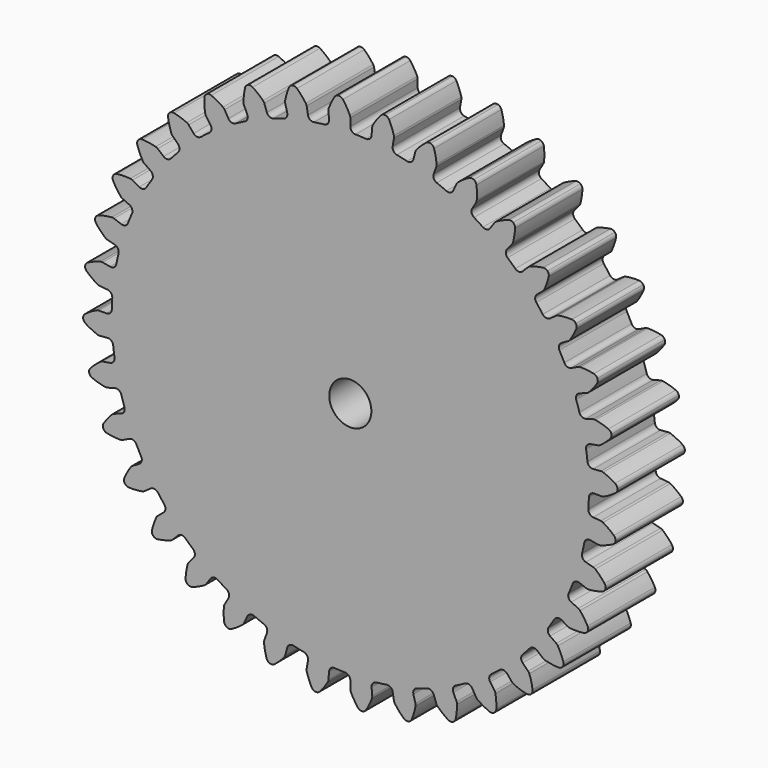
from build123d import *

# Parameters (mm, degrees)
F0_R     = 3.175
F1_DEPTH = 12.7


# Not quite as in the source:
# - ends of sketch curves that miss each other by under 0.0002 mm in the source are joined


with BuildPart() as f1:
    # F0 (on Front) → F1 (new body)
    with BuildSketch(Plane.XZ):
        with BuildLine():
            ThreePointArc((-3.2042183364, 36.6243831745), (-3.3814286726, 36.051583162), (-3.9087160554, 35.7661512552))
            ThreePointArc((-3.9087160554, 35.7661512552), (-4.6962149225, 35.6712938119), (-5.4814313293, 35.5590993614))
            ThreePointArc((-5.4814313293, 35.5590993614), (-6.0646270438, 35.6983333949), (-6.3840506365, 36.2057503103))
            Line((-6.3840506365, 36.2057503103), (-6.5860311993, 37.3512390039))
            ThreePointArc((-6.5860311993, 37.3512390039), (-6.634615599, 37.5176976448), (-6.7181878779, 37.6696338066))
            ThreePointArc((-6.7181878779, 37.6696338066), (-7.3438117619, 38.466585852), (-8.0505487137, 39.1925753064))
            ThreePointArc((-8.0505487137, 39.1925753064), (-8.3662011151, 39.3676879642), (-8.7270294051, 39.3778774973))
            ThreePointArc((-8.7270294051, 39.3778774973), (-8.7297356308, 39.3772929981), (-8.7324354314, 39.3766790101))
            ThreePointArc((-8.7324354314, 39.3766790101), (-9.0551506376, 39.2149515322), (-9.26722306, 38.9228450977))
            ThreePointArc((-9.26722306, 38.9228450977), (-9.6009278616, 37.9661952598), (-9.8311291712, 36.9795113367))
            ThreePointArc((-9.8311291712, 36.9795113367), (-9.8426603818, 36.806491239), (-9.8163443401, 36.6350958219))
            Line((-9.8163443401, 36.6350958219), (-9.5152964565, 35.5115698246))
            ThreePointArc((-9.5152964565, 35.5115698246), (-9.5903488911, 34.9166996794), (-10.0600608633, 34.5440416315))
            ThreePointArc((-10.0600608633, 34.5440416315), (-10.8191240309, 34.3138775427), (-11.5729288743, 34.0670361799))
            ThreePointArc((-11.5729288743, 34.0670361799), (-12.1714422717, 34.1028840626), (-12.5741251249, 34.54712485))
            Line((-12.5741251249, 34.54712485), (-12.9719491733, 35.6401374398))
            ThreePointArc((-12.9719491733, 35.6401374398), (-13.0487007064, 35.7956306075), (-13.1573867722, 35.9307463436))
            ThreePointArc((-13.1573867722, 35.9307463436), (-13.911895294, 36.6069524494), (-14.7339620693, 37.1991889089))
            ThreePointArc((-14.7339620693, 37.1991889089), (-15.0752269954, 37.3168287477), (-15.4323428867, 37.2642063038))
            ThreePointArc((-15.4323428867, 37.2642063038), (-15.4349065016, 37.2631607534), (-15.4374586682, 37.2620872777))
            ThreePointArc((-15.4374586682, 37.2620872777), (-15.7271874235, 37.0467778962), (-15.8853142392, 36.7222832251))
            ThreePointArc((-15.8853142392, 36.7222832251), (-16.047828814, 35.7222198171), (-16.1031969833, 34.710551802))
            ThreePointArc((-16.1031969833, 34.710551802), (-16.0845083842, 34.5381578946), (-16.0288296405, 34.3739360918))
            Line((-16.0288296405, 34.3739360918), (-15.5372571087, 33.3197553953))
            ThreePointArc((-15.5372571087, 33.3197553953), (-15.5078712115, 32.7208899458), (-15.9057358125, 32.2723287829))
            ThreePointArc((-15.9057358125, 32.2723287829), (-16.6132995304, 31.913851468), (-17.3127888316, 31.5398633428))
            ThreePointArc((-17.3127888316, 31.5398633428), (-17.9084343851, 31.4712358548), (-18.3821411842, 31.8388024829))
            Line((-18.3821411842, 31.8388024829), (-18.9637210357, 32.8461283345))
            ThreePointArc((-18.9637210357, 32.8461283345), (-19.0663076459, 32.9859314476), (-19.1968051274, 33.1001213348))
            ThreePointArc((-19.1968051274, 33.1001213348), (-20.0572729274, 33.6350353206), (-20.9696914432, 34.0755239801))
            ThreePointArc((-20.9696914432, 34.0755239801), (-21.3261997318, 34.1321165729), (-21.6687524388, 34.0182810585))
            ThreePointArc((-21.6687524388, 34.0182810585), (-21.6710955487, 34.0168062252), (-21.6734225351, 34.015305879))
            ThreePointArc((-21.6734225351, 34.015305879), (-21.9213615778, 33.7529566604), (-22.0207381836, 33.4059333591))
            ThreePointArc((-22.0207381836, 33.4059333591), (-22.0071246085, 32.3928428016), (-21.8859773037, 31.3869297152))
            ThreePointArc((-21.8859773037, 31.3869297152), (-21.8376367385, 31.2204000998), (-21.7542870633, 31.0683417075))
            Line((-21.7542870633, 31.0683417075), (-21.0871260658, 30.1155370589))
            ThreePointArc((-21.0871260658, 30.1155370589), (-20.9541947126, 29.5308725287), (-21.2681230277, 29.0200375549))
            ThreePointArc((-21.2681230277, 29.0200375549), (-21.9026883304, 28.5441391657), (-22.526608461, 28.054367718))
            ThreePointArc((-22.526608461, 28.054367718), (-23.1012877819, 27.8833500709), (-23.6316251854, 28.1630742135))
            Line((-23.6316251854, 28.1630742135), (-24.3792898306, 29.0541062406))
            ThreePointArc((-24.3792898306, 29.0541062406), (-24.5045944755, 29.1739714524), (-24.6529382729, 29.2637658888))
            ThreePointArc((-24.6529382729, 29.2637658888), (-25.5932204724, 29.6411346638), (-26.5682673537, 29.9164914982))
            ThreePointArc((-26.5682673537, 29.9164914982), (-26.929186681, 29.9103173077), (-27.246767913, 29.7387275572))
            ThreePointArc((-27.246767913, 29.7387275572), (-27.2488193237, 29.7368682532), (-27.2508504255, 29.7349866237))
            ThreePointArc((-27.2508504255, 29.7349866237), (-27.4494662534, 29.4335689163), (-27.4870731413, 29.0745611122))
            ThreePointArc((-27.4870731413, 29.0745611122), (-27.2977450579, 28.0792256492), (-27.0037632785, 27.1096316515))
            ThreePointArc((-27.0037632785, 27.1096316515), (-26.9272395509, 26.9540262462), (-26.8187514818, 26.8187514818))
            Line((-26.8187514818, 26.8187514818), (-25.9962733681, 25.9962733681))
            ThreePointArc((-25.9962733681, 25.9962733681), (-25.7638356106, 25.4435744931), (-25.984289087, 24.8859871706))
            ThreePointArc((-25.984289087, 24.8859871706), (-26.5265750288, 24.3071276388), (-27.0559684913, 23.7164543263))
            ThreePointArc((-27.0559684913, 23.7164543263), (-27.5922202392, 23.4482428047), (-28.1630742135, 23.6316251854))
            Line((-28.1630742135, 23.6316251854), (-29.0541062406, 24.3792898306))
            ThreePointArc((-29.0541062406, 24.3792898306), (-29.1983216019, 24.4755750974), (-29.360004364, 24.5382457244))
            ThreePointArc((-29.360004364, 24.5382457244), (-30.3515309641, 24.7466031293), (-31.3595799049, 24.8484615606))
            ThreePointArc((-31.3595799049, 24.8484615606), (-31.7139439196, 24.7797081865), (-31.9969041317, 24.5555778676))
            ThreePointArc((-31.9969041317, 24.5555778676), (-31.9986015121, 24.5533905869), (-32.0002750154, 24.5511848465))
            ThreePointArc((-32.0002750154, 24.5511848465), (-32.1435327869, 24.2198570747), (-32.1182272908, 23.8597730383))
            ThreePointArc((-32.1182272908, 23.8597730383), (-31.7589373371, 22.9124354342), (-31.3010535707, 22.0086211482))
            ThreePointArc((-31.3010535707, 22.0086211482), (-31.1986718154, 21.8686679446), (-31.0683417075, 21.7542870633))
            Line((-31.0683417075, 21.7542870633), (-30.1155370589, 21.0871260658))
            ThreePointArc((-30.1155370589, 21.0871260658), (-29.7906554007, 20.5831863217), (-29.910935671, 19.995788659))
            ThreePointArc((-29.910935671, 19.995788659), (-30.344465168, 19.3315563387), (-30.7632466099, 18.6579284709))
            ThreePointArc((-30.7632466099, 18.6579284709), (-31.2447770469, 18.3006725462), (-31.8388024829, 18.3821411842))
            Line((-31.8388024829, 18.3821411842), (-32.8461283345, 18.9637210357))
            ThreePointArc((-32.8461283345, 18.9637210357), (-33.0048725015, 19.0335007782), (-33.1749815793, 19.0671433806))
            ThreePointArc((-33.1749815793, 19.0671433806), (-34.1876255461, 19.1001585812), (-35.1980474894, 19.0254236925))
            ThreePointArc((-35.1980474894, 19.0254236925), (-35.5350890203, 18.8961801711), (-35.7748306096, 18.6263193703))
            ThreePointArc((-35.7748306096, 18.6263193703), (-35.7761223856, 18.6238705723), (-35.7773874418, 18.6214077412))
            ThreePointArc((-35.7773874418, 18.6214077412), (-35.8609343421, 18.2702371318), (-35.7734853566, 17.9200178343))
            ThreePointArc((-35.7734853566, 17.9200178343), (-35.255150376, 17.0494624628), (-34.6472771892, 16.2388898283))
            ThreePointArc((-34.6472771892, 16.2388898283), (-34.5221482241, 16.1188412335), (-34.3739360918, 16.0288296405))
            Line((-34.3739360918, 16.0288296405), (-33.3197553953, 15.5372571087))
            ThreePointArc((-33.3197553953, 15.5372571087), (-32.9123012013, 15.0973884495), (-32.9287536103, 14.4980282274))
            ThreePointArc((-32.9287536103, 14.4980282274), (-33.2403540882, 13.7686054814), (-33.5357990473, 13.0324909004))
            ThreePointArc((-33.5357990473, 13.0324909004), (-33.9479771147, 12.597045613), (-34.54712485, 12.5741251249))
            Line((-34.54712485, 12.5741251249), (-35.6401374398, 12.9719491733))
            ThreePointArc((-35.6401374398, 12.9719491733), (-35.8085870514, 13.0131031693), (-35.9819537667, 13.0166955336))
            ThreePointArc((-35.9819537667, 13.0166955336), (-36.9849464257, 12.8733653796), (-37.967040212, 12.6243079527))
            ThreePointArc((-37.967040212, 12.6243079527), (-38.2765184228, 12.4385012832), (-38.4657569623, 12.1311095843))
            ThreePointArc((-38.4657569623, 12.1311095843), (-38.4666038841, 12.1284736744), (-38.4674220551, 12.1258285845))
            ThreePointArc((-38.4674220551, 12.1258285845), (-38.4887195539, 11.7654852788), (-38.3417841721, 11.4357719564))
            ThreePointArc((-38.3417841721, 11.4357719564), (-37.6801535108, 10.6684502019), (-36.9407608227, 9.9757480582))
            ThreePointArc((-36.9407608227, 9.9757480582), (-36.796686628, 9.879251688), (-36.6350958219, 9.8163443401))
            Line((-36.6350958219, 9.8163443401), (-35.5115698246, 9.5152964565))
            ThreePointArc((-35.5115698246, 9.5152964565), (-35.0339233843, 9.1528640689), (-34.9460480339, 8.5597525445))
            ThreePointArc((-34.9460480339, 8.5597525445), (-35.1262516698, 7.7873025138), (-35.2893832006, 7.0110676886))
            ThreePointArc((-35.2893832006, 7.0110676886), (-35.6196850763, 6.5106638233), (-36.2057503103, 6.3840506365))
            Line((-36.2057503103, 6.3840506365), (-37.3512390039, 6.5860311993))
            ThreePointArc((-37.3512390039, 6.5860311993), (-37.5242758038, 6.5973090056), (-37.6956324966, 6.5707419796))
            ThreePointArc((-37.6956324966, 6.5707419796), (-38.6584984233, 6.2554214853), (-39.58242363, 5.839609004))
            ThreePointArc((-39.58242363, 5.839609004), (-39.8549351818, 5.602884828), (-39.9879207543, 5.2673021721))
            ThreePointArc((-39.9879207543, 5.2673021721), (-39.9882970885, 5.2645592413), (-39.9886435147, 5.2618122623))
            ThreePointArc((-39.9886435147, 5.2618122623), (-39.9470444982, 4.9032451093), (-39.7450872775, 4.6040559343))
            ThreePointArc((-39.7450872775, 4.6040559343), (-38.9602642482, 3.9632824801), (-38.1118181316, 3.4094982313))
            ThreePointArc((-38.1118181316, 3.4094982313), (-37.9531763288, 3.3394860792), (-37.7831167038, 3.3055943843))
            Line((-37.7831167038, 3.3055943843), (-36.6243831745, 3.2042183364))
            ThreePointArc((-36.6243831745, 3.2042183364), (-36.0910575332, 2.9302345451), (-35.9015244715, 2.3613931119))
            ThreePointArc((-35.9015244715, 2.3613931119), (-35.9448558691, 1.5693863), (-35.9707173026, 0.7766167329))
            ThreePointArc((-35.9707173026, 0.7766167329), (-36.2091069313, 0.2264588079), (-36.7642823684, 0))
            Line((-36.7642823684, 0), (-37.9274420715, 0))
            ThreePointArc((-37.9274420715, 0), (-38.0998084241, -0.0189410539), (-38.263948508, -0.0748602444))
            ThreePointArc((-38.263948508, -0.0748602444), (-39.1574315086, -0.5525902255), (-39.9951151356, -1.1225235092))
            ThreePointArc((-39.9951151356, -1.1225235092), (-40.2223799029, -1.4029724475), (-40.2950718091, -1.7565495511))
            ThreePointArc((-40.2950718091, -1.7565495511), (-40.294966121, -1.7593161604), (-40.2948302763, -1.7620815628))
            ThreePointArc((-40.2948302763, -1.7620815628), (-40.1915987096, -2.1079776817), (-39.9407560179, -2.3675519975))
            ThreePointArc((-39.9407560179, -2.3675519975), (-39.0565870713, -2.8623075744), (-38.124867132, -3.2603474741))
            ThreePointArc((-38.124867132, -3.2603474741), (-37.956477972, -3.3017481243), (-37.7831167038, -3.3055943843))
            Line((-37.7831167038, -3.3055943843), (-36.6243831745, -3.2042183364))
            ThreePointArc((-36.6243831745, -3.2042183364), (-36.051583162, -3.3814286726), (-35.7661512552, -3.9087160554))
            ThreePointArc((-35.7661512552, -3.9087160554), (-35.6712938119, -4.6962149225), (-35.5590993614, -5.4814313293))
            ThreePointArc((-35.5590993614, -5.4814313293), (-35.6983333949, -6.0646270438), (-36.2057503103, -6.3840506365))
            Line((-36.2057503103, -6.3840506365), (-37.3512390039, -6.5860311993))
            ThreePointArc((-37.3512390039, -6.5860311993), (-37.5176976448, -6.634615599), (-37.6696338066, -6.7181878779))
            ThreePointArc((-37.6696338066, -6.7181878779), (-38.466585852, -7.3438117619), (-39.1925753064, -8.0505487137))
            ThreePointArc((-39.1925753064, -8.0505487137), (-39.3676879642, -8.3662011151), (-39.3778774973, -8.7270294051))
            ThreePointArc((-39.3778774973, -8.7270294051), (-39.3772929981, -8.7297356308), (-39.3766790101, -8.7324354314))
            ThreePointArc((-39.3766790101, -8.7324354314), (-39.2149515322, -9.0551506376), (-38.9228450977, -9.26722306))
            ThreePointArc((-38.9228450977, -9.26722306), (-37.9661952598, -9.6009278616), (-36.9795113367, -9.8311291712))
            ThreePointArc((-36.9795113367, -9.8311291712), (-36.806491239, -9.8426603818), (-36.6350958219, -9.8163443401))
            Line((-36.6350958219, -9.8163443401), (-35.5115698246, -9.5152964565))
            ThreePointArc((-35.5115698246, -9.5152964565), (-34.9166996794, -9.5903488911), (-34.5440416315, -10.0600608633))
            ThreePointArc((-34.5440416315, -10.0600608633), (-34.3138775427, -10.8191240309), (-34.0670361799, -11.5729288743))
            ThreePointArc((-34.0670361799, -11.5729288743), (-34.1028840626, -12.1714422717), (-34.54712485, -12.5741251249))
            Line((-34.54712485, -12.5741251249), (-35.6401374398, -12.9719491733))
            ThreePointArc((-35.6401374398, -12.9719491733), (-35.7956306075, -13.0487007064), (-35.9307463436, -13.1573867722))
            ThreePointArc((-35.9307463436, -13.1573867722), (-36.6069524494, -13.911895294), (-37.1991889089, -14.7339620693))
            ThreePointArc((-37.1991889089, -14.7339620693), (-37.3168287477, -15.0752269954), (-37.2642063038, -15.4323428867))
            ThreePointArc((-37.2642063038, -15.4323428867), (-37.2631607534, -15.4349065016), (-37.2620872777, -15.4374586682))
            ThreePointArc((-37.2620872777, -15.4374586682), (-37.0467778962, -15.7271874235), (-36.7222832251, -15.8853142392))
            ThreePointArc((-36.7222832251, -15.8853142392), (-35.7222198171, -16.047828814), (-34.710551802, -16.1031969833))
            ThreePointArc((-34.710551802, -16.1031969833), (-34.5381578946, -16.0845083842), (-34.3739360918, -16.0288296405))
            Line((-34.3739360918, -16.0288296405), (-33.3197553953, -15.5372571087))
            ThreePointArc((-33.3197553953, -15.5372571087), (-32.7208899458, -15.5078712115), (-32.2723287829, -15.9057358125))
            ThreePointArc((-32.2723287829, -15.9057358125), (-31.913851468, -16.6132995304), (-31.5398633428, -17.3127888316))
            ThreePointArc((-31.5398633428, -17.3127888316), (-31.4712358548, -17.9084343851), (-31.8388024829, -18.3821411842))
            Line((-31.8388024829, -18.3821411842), (-32.8461283345, -18.9637210357))
            ThreePointArc((-32.8461283345, -18.9637210357), (-32.9859314476, -19.0663076459), (-33.1001213348, -19.1968051274))
            ThreePointArc((-33.1001213348, -19.1968051274), (-33.6350353206, -20.0572729274), (-34.0755239801, -20.9696914432))
            ThreePointArc((-34.0755239801, -20.9696914432), (-34.1321165729, -21.3261997318), (-34.0182810585, -21.6687524388))
            ThreePointArc((-34.0182810585, -21.6687524388), (-34.0168062252, -21.6710955487), (-34.015305879, -21.6734225351))
            ThreePointArc((-34.015305879, -21.6734225351), (-33.7529566604, -21.9213615778), (-33.4059333591, -22.0207381836))
            ThreePointArc((-33.4059333591, -22.0207381836), (-32.3928428016, -22.0071246085), (-31.3869297152, -21.8859773037))
            ThreePointArc((-31.3869297152, -21.8859773037), (-31.2204000998, -21.8376367385), (-31.0683417075, -21.7542870633))
            Line((-31.0683417075, -21.7542870633), (-30.1155370589, -21.0871260658))
            ThreePointArc((-30.1155370589, -21.0871260658), (-29.5308725287, -20.9541947126), (-29.0200375549, -21.2681230277))
            ThreePointArc((-29.0200375549, -21.2681230277), (-28.5441391657, -21.9026883304), (-28.054367718, -22.526608461))
            ThreePointArc((-28.054367718, -22.526608461), (-27.8833500709, -23.1012877819), (-28.1630742135, -23.6316251854))
            Line((-28.1630742135, -23.6316251854), (-29.0541062406, -24.3792898306))
            ThreePointArc((-29.0541062406, -24.3792898306), (-29.1739714524, -24.5045944755), (-29.2637658888, -24.6529382729))
            ThreePointArc((-29.2637658888, -24.6529382729), (-29.6411346638, -25.5932204724), (-29.9164914982, -26.5682673537))
            ThreePointArc((-29.9164914982, -26.5682673537), (-29.9103173077, -26.929186681), (-29.7387275572, -27.246767913))
            ThreePointArc((-29.7387275572, -27.246767913), (-29.7368682532, -27.2488193237), (-29.7349866237, -27.2508504255))
            ThreePointArc((-29.7349866237, -27.2508504255), (-29.4335689163, -27.4494662534), (-29.0745611122, -27.4870731413))
            ThreePointArc((-29.0745611122, -27.4870731413), (-28.0792256492, -27.2977450579), (-27.1096316515, -27.0037632785))
            ThreePointArc((-27.1096316515, -27.0037632785), (-26.9540262462, -26.9272395509), (-26.8187514818, -26.8187514818))
            Line((-26.8187514818, -26.8187514818), (-25.9962733681, -25.9962733681))
            ThreePointArc((-25.9962733681, -25.9962733681), (-25.4435744931, -25.7638356106), (-24.8859871706, -25.984289087))
            ThreePointArc((-24.8859871706, -25.984289087), (-24.3071276388, -26.5265750288), (-23.7164543263, -27.0559684913))
            ThreePointArc((-23.7164543263, -27.0559684913), (-23.4482428047, -27.5922202392), (-23.6316251854, -28.1630742135))
            Line((-23.6316251854, -28.1630742135), (-24.3792898306, -29.0541062406))
            ThreePointArc((-24.3792898306, -29.0541062406), (-24.4755750974, -29.1983216019), (-24.5382457244, -29.360004364))
            ThreePointArc((-24.5382457244, -29.360004364), (-24.7466031293, -30.3515309641), (-24.8484615606, -31.3595799049))
            ThreePointArc((-24.8484615606, -31.3595799049), (-24.7797081865, -31.7139439196), (-24.5555778676, -31.9969041317))
            ThreePointArc((-24.5555778676, -31.9969041317), (-24.5533905869, -31.9986015121), (-24.5511848465, -32.0002750154))
            ThreePointArc((-24.5511848465, -32.0002750154), (-24.2198570747, -32.1435327869), (-23.8597730383, -32.1182272908))
            ThreePointArc((-23.8597730383, -32.1182272908), (-22.9124354342, -31.7589373371), (-22.0086211482, -31.3010535707))
            ThreePointArc((-22.0086211482, -31.3010535707), (-21.8686679446, -31.1986718154), (-21.7542870633, -31.0683417075))
            Line((-21.7542870633, -31.0683417075), (-21.0871260658, -30.1155370589))
            ThreePointArc((-21.0871260658, -30.1155370589), (-20.5831863217, -29.7906554007), (-19.995788659, -29.910935671))
            ThreePointArc((-19.995788659, -29.910935671), (-19.3315563387, -30.344465168), (-18.6579284709, -30.7632466099))
            ThreePointArc((-18.6579284709, -30.7632466099), (-18.3006725462, -31.2447770469), (-18.3821411842, -31.8388024829))
            Line((-18.3821411842, -31.8388024829), (-18.9637210357, -32.8461283345))
            ThreePointArc((-18.9637210357, -32.8461283345), (-19.0335007782, -33.0048725015), (-19.0671433806, -33.1749815793))
            ThreePointArc((-19.0671433806, -33.1749815793), (-19.1001585812, -34.1876255461), (-19.0254236925, -35.1980474894))
            ThreePointArc((-19.0254236925, -35.1980474894), (-18.8961801711, -35.5350890203), (-18.6263193703, -35.7748306096))
            ThreePointArc((-18.6263193703, -35.7748306096), (-18.6238705723, -35.7761223856), (-18.6214077412, -35.7773874418))
            ThreePointArc((-18.6214077412, -35.7773874418), (-18.2702371318, -35.8609343421), (-17.9200178343, -35.7734853566))
            ThreePointArc((-17.9200178343, -35.7734853566), (-17.0494624628, -35.255150376), (-16.2388898283, -34.6472771892))
            ThreePointArc((-16.2388898283, -34.6472771892), (-16.1188412335, -34.5221482241), (-16.0288296405, -34.3739360918))
            Line((-16.0288296405, -34.3739360918), (-15.5372571087, -33.3197553953))
            ThreePointArc((-15.5372571087, -33.3197553953), (-15.0973884495, -32.9123012013), (-14.4980282274, -32.9287536103))
            ThreePointArc((-14.4980282274, -32.9287536103), (-13.7686054814, -33.2403540882), (-13.0324909004, -33.5357990473))
            ThreePointArc((-13.0324909004, -33.5357990473), (-12.597045613, -33.9479771147), (-12.5741251249, -34.54712485))
            Line((-12.5741251249, -34.54712485), (-12.9719491733, -35.6401374398))
            ThreePointArc((-12.9719491733, -35.6401374398), (-13.0131031693, -35.8085870514), (-13.0166955336, -35.9819537667))
            ThreePointArc((-13.0166955336, -35.9819537667), (-12.8733653796, -36.9849464257), (-12.6243079527, -37.967040212))
            ThreePointArc((-12.6243079527, -37.967040212), (-12.4385012832, -38.2765184228), (-12.1311095843, -38.4657569623))
            ThreePointArc((-12.1311095843, -38.4657569623), (-12.1284736744, -38.4666038841), (-12.1258285845, -38.4674220551))
            ThreePointArc((-12.1258285845, -38.4674220551), (-11.7654852788, -38.4887195539), (-11.4357719564, -38.3417841721))
            ThreePointArc((-11.4357719564, -38.3417841721), (-10.6684502019, -37.6801535108), (-9.9757480582, -36.9407608227))
            ThreePointArc((-9.9757480582, -36.9407608227), (-9.879251688, -36.796686628), (-9.8163443401, -36.6350958219))
            Line((-9.8163443401, -36.6350958219), (-9.5152964565, -35.5115698246))
            ThreePointArc((-9.5152964565, -35.5115698246), (-9.1528640689, -35.0339233843), (-8.5597525445, -34.9460480339))
            ThreePointArc((-8.5597525445, -34.9460480339), (-7.7873025138, -35.1262516698), (-7.0110676886, -35.2893832006))
            ThreePointArc((-7.0110676886, -35.2893832006), (-6.5106638233, -35.6196850763), (-6.3840506365, -36.2057503103))
            Line((-6.3840506365, -36.2057503103), (-6.5860311993, -37.3512390039))
            ThreePointArc((-6.5860311993, -37.3512390039), (-6.5973090056, -37.5242758038), (-6.5707419796, -37.6956324966))
            ThreePointArc((-6.5707419796, -37.6956324966), (-6.2554214853, -38.6584984233), (-5.839609004, -39.58242363))
            ThreePointArc((-5.839609004, -39.58242363), (-5.602884828, -39.8549351818), (-5.2673021721, -39.9879207543))
            ThreePointArc((-5.2673021721, -39.9879207543), (-5.2645592413, -39.9882970885), (-5.2618122623, -39.9886435147))
            ThreePointArc((-5.2618122623, -39.9886435147), (-4.9032451093, -39.9470444982), (-4.6040559343, -39.7450872775))
            ThreePointArc((-4.6040559343, -39.7450872775), (-3.9632824801, -38.9602642482), (-3.4094982313, -38.1118181316))
            ThreePointArc((-3.4094982313, -38.1118181316), (-3.3394860792, -37.9531763288), (-3.3055943843, -37.7831167038))
            Line((-3.3055943843, -37.7831167038), (-3.2042183364, -36.6243831745))
            ThreePointArc((-3.2042183364, -36.6243831745), (-2.9302345451, -36.0910575332), (-2.3613931119, -35.9015244715))
            ThreePointArc((-2.3613931119, -35.9015244715), (-1.5693863, -35.9448558691), (-0.7766167329, -35.9707173026))
            ThreePointArc((-0.7766167329, -35.9707173026), (-0.2264588079, -36.2091069313), (0, -36.7642823684))
            Line((0, -36.7642823684), (0, -37.9274420715))
            ThreePointArc((0, -37.9274420715), (0.0189410539, -38.0998084241), (0.0748602444, -38.263948508))
            ThreePointArc((0.0748602444, -38.263948508), (0.5525902255, -39.1574315086), (1.1225235092, -39.9951151356))
            ThreePointArc((1.1225235092, -39.9951151356), (1.4029724475, -40.2223799029), (1.7565495511, -40.2950718091))
            ThreePointArc((1.7565495511, -40.2950718091), (1.7593161604, -40.294966121), (1.7620815628, -40.2948302763))
            ThreePointArc((1.7620815628, -40.2948302763), (2.1079776817, -40.1915987096), (2.3675519975, -39.9407560179))
            ThreePointArc((2.3675519975, -39.9407560179), (2.8623075744, -39.0565870713), (3.2603474741, -38.124867132))
            ThreePointArc((3.2603474741, -38.124867132), (3.3017481243, -37.956477972), (3.3055943843, -37.7831167038))
            Line((3.3055943843, -37.7831167038), (3.2042183364, -36.6243831745))
            ThreePointArc((3.2042183364, -36.6243831745), (3.3814286726, -36.051583162), (3.9087160554, -35.7661512552))
            ThreePointArc((3.9087160554, -35.7661512552), (4.6962149225, -35.6712938119), (5.4814313293, -35.5590993614))
            ThreePointArc((5.4814313293, -35.5590993614), (6.0646270438, -35.6983333949), (6.3840506365, -36.2057503103))
            Line((6.3840506365, -36.2057503103), (6.5860311993, -37.3512390039))
            ThreePointArc((6.5860311993, -37.3512390039), (6.634615599, -37.5176976448), (6.7181878779, -37.6696338066))
            ThreePointArc((6.7181878779, -37.6696338066), (7.3438117619, -38.466585852), (8.0505487137, -39.1925753064))
            ThreePointArc((8.0505487137, -39.1925753064), (8.3662011151, -39.3676879642), (8.7270294051, -39.3778774973))
            ThreePointArc((8.7270294051, -39.3778774973), (8.7297356308, -39.3772929981), (8.7324354314, -39.3766790101))
            ThreePointArc((8.7324354314, -39.3766790101), (9.0551506376, -39.2149515322), (9.26722306, -38.9228450977))
            ThreePointArc((9.26722306, -38.9228450977), (9.6009278616, -37.9661952598), (9.8311291712, -36.9795113367))
            ThreePointArc((9.8311291712, -36.9795113367), (9.8426603818, -36.806491239), (9.8163443401, -36.6350958219))
            Line((9.8163443401, -36.6350958219), (9.5152964565, -35.5115698246))
            ThreePointArc((9.5152964565, -35.5115698246), (9.5903488911, -34.9166996794), (10.0600608633, -34.5440416315))
            ThreePointArc((10.0600608633, -34.5440416315), (10.8191240309, -34.3138775427), (11.5729288743, -34.0670361799))
            ThreePointArc((11.5729288743, -34.0670361799), (12.1714422717, -34.1028840626), (12.5741251249, -34.54712485))
            Line((12.5741251249, -34.54712485), (12.9719491733, -35.6401374398))
            ThreePointArc((12.9719491733, -35.6401374398), (13.0487007064, -35.7956306075), (13.1573867722, -35.9307463436))
            ThreePointArc((13.1573867722, -35.9307463436), (13.911895294, -36.6069524494), (14.7339620693, -37.1991889089))
            ThreePointArc((14.7339620693, -37.1991889089), (15.0752269954, -37.3168287477), (15.4323428867, -37.2642063038))
            ThreePointArc((15.4323428867, -37.2642063038), (15.4349065016, -37.2631607534), (15.4374586682, -37.2620872777))
            ThreePointArc((15.4374586682, -37.2620872777), (15.7271874235, -37.0467778962), (15.8853142392, -36.7222832251))
            ThreePointArc((15.8853142392, -36.7222832251), (16.047828814, -35.7222198171), (16.1031969833, -34.710551802))
            ThreePointArc((16.1031969833, -34.710551802), (16.0845083842, -34.5381578946), (16.0288296405, -34.3739360918))
            Line((16.0288296405, -34.3739360918), (15.5372571087, -33.3197553953))
            ThreePointArc((15.5372571087, -33.3197553953), (15.5078712115, -32.7208899458), (15.9057358125, -32.2723287829))
            ThreePointArc((15.9057358125, -32.2723287829), (16.6132995304, -31.913851468), (17.3127888316, -31.5398633428))
            ThreePointArc((17.3127888316, -31.5398633428), (17.9084343851, -31.4712358548), (18.3821411842, -31.8388024829))
            Line((18.3821411842, -31.8388024829), (18.9637210357, -32.8461283345))
            ThreePointArc((18.9637210357, -32.8461283345), (19.0663076459, -32.9859314476), (19.1968051274, -33.1001213348))
            ThreePointArc((19.1968051274, -33.1001213348), (20.0572729274, -33.6350353206), (20.9696914432, -34.0755239801))
            ThreePointArc((20.9696914432, -34.0755239801), (21.3261997318, -34.1321165729), (21.6687524388, -34.0182810585))
            ThreePointArc((21.6687524388, -34.0182810585), (21.6710955487, -34.0168062252), (21.6734225351, -34.015305879))
            ThreePointArc((21.6734225351, -34.015305879), (21.9213615778, -33.7529566604), (22.0207381836, -33.4059333591))
            ThreePointArc((22.0207381836, -33.4059333591), (22.0071246085, -32.3928428016), (21.8859773037, -31.3869297152))
            ThreePointArc((21.8859773037, -31.3869297152), (21.8376367385, -31.2204000998), (21.7542870633, -31.0683417075))
            Line((21.7542870633, -31.0683417075), (21.0871260658, -30.1155370589))
            ThreePointArc((21.0871260658, -30.1155370589), (20.9541947126, -29.5308725287), (21.2681230277, -29.0200375549))
            ThreePointArc((21.2681230277, -29.0200375549), (21.9026883304, -28.5441391657), (22.526608461, -28.054367718))
            ThreePointArc((22.526608461, -28.054367718), (23.1012877819, -27.8833500709), (23.6316251854, -28.1630742135))
            Line((23.6316251854, -28.1630742135), (24.3792898306, -29.0541062406))
            ThreePointArc((24.3792898306, -29.0541062406), (24.5045944755, -29.1739714524), (24.6529382729, -29.2637658888))
            ThreePointArc((24.6529382729, -29.2637658888), (25.5932204724, -29.6411346638), (26.5682673537, -29.9164914982))
            ThreePointArc((26.5682673537, -29.9164914982), (26.929186681, -29.9103173077), (27.246767913, -29.7387275572))
            ThreePointArc((27.246767913, -29.7387275572), (27.2488193237, -29.7368682532), (27.2508504255, -29.7349866237))
            ThreePointArc((27.2508504255, -29.7349866237), (27.4494662534, -29.4335689163), (27.4870731413, -29.0745611122))
            ThreePointArc((27.4870731413, -29.0745611122), (27.2977450579, -28.0792256492), (27.0037632785, -27.1096316515))
            ThreePointArc((27.0037632785, -27.1096316515), (26.9272395509, -26.9540262462), (26.8187514818, -26.8187514818))
            Line((26.8187514818, -26.8187514818), (25.9962733681, -25.9962733681))
            ThreePointArc((25.9962733681, -25.9962733681), (25.7638356106, -25.4435744931), (25.984289087, -24.8859871706))
            ThreePointArc((25.984289087, -24.8859871706), (26.5265750288, -24.3071276388), (27.0559684913, -23.7164543263))
            ThreePointArc((27.0559684913, -23.7164543263), (27.5922202392, -23.4482428047), (28.1630742135, -23.6316251854))
            Line((28.1630742135, -23.6316251854), (29.0541062406, -24.3792898306))
            ThreePointArc((29.0541062406, -24.3792898306), (29.1983216019, -24.4755750974), (29.360004364, -24.5382457244))
            ThreePointArc((29.360004364, -24.5382457244), (30.3515309641, -24.7466031293), (31.3595799049, -24.8484615606))
            ThreePointArc((31.3595799049, -24.8484615606), (31.7139439196, -24.7797081865), (31.9969041317, -24.5555778676))
            ThreePointArc((31.9969041317, -24.5555778676), (31.9986015121, -24.5533905869), (32.0002750154, -24.5511848465))
            ThreePointArc((32.0002750154, -24.5511848465), (32.1435327869, -24.2198570747), (32.1182272908, -23.8597730383))
            ThreePointArc((32.1182272908, -23.8597730383), (31.7589373371, -22.9124354342), (31.3010535707, -22.0086211482))
            ThreePointArc((31.3010535707, -22.0086211482), (31.1986718154, -21.8686679446), (31.0683417075, -21.7542870633))
            Line((31.0683417075, -21.7542870633), (30.1155370589, -21.0871260658))
            ThreePointArc((30.1155370589, -21.0871260658), (29.7906554007, -20.5831863217), (29.910935671, -19.995788659))
            ThreePointArc((29.910935671, -19.995788659), (30.344465168, -19.3315563387), (30.7632466099, -18.6579284709))
            ThreePointArc((30.7632466099, -18.6579284709), (31.2447770469, -18.3006725462), (31.8388024829, -18.3821411842))
            Line((31.8388024829, -18.3821411842), (32.8461283345, -18.9637210357))
            ThreePointArc((32.8461283345, -18.9637210357), (33.0048725015, -19.0335007782), (33.1749815793, -19.0671433806))
            ThreePointArc((33.1749815793, -19.0671433806), (34.1876255461, -19.1001585812), (35.1980474894, -19.0254236925))
            ThreePointArc((35.1980474894, -19.0254236925), (35.5350890203, -18.8961801711), (35.7748306096, -18.6263193703))
            ThreePointArc((35.7748306096, -18.6263193703), (35.7761223856, -18.6238705723), (35.7773874418, -18.6214077412))
            ThreePointArc((35.7773874418, -18.6214077412), (35.8609343421, -18.2702371318), (35.7734853566, -17.9200178343))
            ThreePointArc((35.7734853566, -17.9200178343), (35.255150376, -17.0494624628), (34.6472771892, -16.2388898283))
            ThreePointArc((34.6472771892, -16.2388898283), (34.5221482241, -16.1188412335), (34.3739360918, -16.0288296405))
            Line((34.3739360918, -16.0288296405), (33.3197553953, -15.5372571087))
            ThreePointArc((33.3197553953, -15.5372571087), (32.9123012013, -15.0973884495), (32.9287536103, -14.4980282274))
            ThreePointArc((32.9287536103, -14.4980282274), (33.2403540882, -13.7686054814), (33.5357990473, -13.0324909004))
            ThreePointArc((33.5357990473, -13.0324909004), (33.9479771147, -12.597045613), (34.54712485, -12.5741251249))
            Line((34.54712485, -12.5741251249), (35.6401374398, -12.9719491733))
            ThreePointArc((35.6401374398, -12.9719491733), (35.8085870514, -13.0131031693), (35.9819537667, -13.0166955336))
            ThreePointArc((35.9819537667, -13.0166955336), (36.9849464257, -12.8733653796), (37.967040212, -12.6243079527))
            ThreePointArc((37.967040212, -12.6243079527), (38.2765184228, -12.4385012832), (38.4657569623, -12.1311095843))
            ThreePointArc((38.4657569623, -12.1311095843), (38.4666038841, -12.1284736744), (38.4674220551, -12.1258285845))
            ThreePointArc((38.4674220551, -12.1258285845), (38.4887195539, -11.7654852788), (38.3417841721, -11.4357719564))
            ThreePointArc((38.3417841721, -11.4357719564), (37.6801535108, -10.6684502019), (36.9407608227, -9.9757480582))
            ThreePointArc((36.9407608227, -9.9757480582), (36.796686628, -9.879251688), (36.6350958219, -9.8163443401))
            Line((36.6350958219, -9.8163443401), (35.5115698246, -9.5152964565))
            ThreePointArc((35.5115698246, -9.5152964565), (35.0339233843, -9.1528640689), (34.9460480339, -8.5597525445))
            ThreePointArc((34.9460480339, -8.5597525445), (35.1262516698, -7.7873025138), (35.2893832006, -7.0110676886))
            ThreePointArc((35.2893832006, -7.0110676886), (35.6196850763, -6.5106638233), (36.2057503103, -6.3840506365))
            Line((36.2057503103, -6.3840506365), (37.3512390039, -6.5860311993))
            ThreePointArc((37.3512390039, -6.5860311993), (37.5242758038, -6.5973090056), (37.6956324966, -6.5707419796))
            ThreePointArc((37.6956324966, -6.5707419796), (38.6584984233, -6.2554214853), (39.58242363, -5.839609004))
            ThreePointArc((39.58242363, -5.839609004), (39.8549351818, -5.602884828), (39.9879207543, -5.2673021721))
            ThreePointArc((39.9879207543, -5.2673021721), (39.9882970885, -5.2645592413), (39.9886435147, -5.2618122623))
            ThreePointArc((39.9886435147, -5.2618122623), (39.9470444982, -4.9032451093), (39.7450872775, -4.6040559343))
            ThreePointArc((39.7450872775, -4.6040559343), (38.9602642482, -3.9632824801), (38.1118181316, -3.4094982313))
            ThreePointArc((38.1118181316, -3.4094982313), (37.9531763288, -3.3394860792), (37.7831167038, -3.3055943843))
            Line((37.7831167038, -3.3055943843), (36.6243831745, -3.2042183364))
            ThreePointArc((36.6243831745, -3.2042183364), (36.0910575332, -2.9302345451), (35.9015244715, -2.3613931119))
            ThreePointArc((35.9015244715, -2.3613931119), (35.9448558691, -1.5693863), (35.9707173026, -0.7766167329))
            ThreePointArc((35.9707173026, -0.7766167329), (36.2091069313, -0.2264588079), (36.7642823684, 0))
            Line((36.7642823684, 0), (37.9274420715, 0))
            ThreePointArc((37.9274420715, 0), (38.0998084241, 0.0189410539), (38.263948508, 0.0748602444))
            ThreePointArc((38.263948508, 0.0748602444), (39.1574315086, 0.5525902255), (39.9951151356, 1.1225235092))
            ThreePointArc((39.9951151356, 1.1225235092), (40.2223799029, 1.4029724475), (40.2950718091, 1.7565495511))
            ThreePointArc((40.2950718091, 1.7565495511), (40.294966121, 1.7593161604), (40.2948302763, 1.7620815628))
            ThreePointArc((40.2948302763, 1.7620815628), (40.1915987096, 2.1079776817), (39.9407560179, 2.3675519975))
            ThreePointArc((39.9407560179, 2.3675519975), (39.0565870713, 2.8623075744), (38.124867132, 3.2603474741))
            ThreePointArc((38.124867132, 3.2603474741), (37.956477972, 3.3017481243), (37.7831167038, 3.3055943843))
            Line((37.7831167038, 3.3055943843), (36.6243831745, 3.2042183364))
            ThreePointArc((36.6243831745, 3.2042183364), (36.051583162, 3.3814286726), (35.7661512552, 3.9087160554))
            ThreePointArc((35.7661512552, 3.9087160554), (35.6712938119, 4.6962149225), (35.5590993614, 5.4814313293))
            ThreePointArc((35.5590993614, 5.4814313293), (35.6983333949, 6.0646270438), (36.2057503103, 6.3840506365))
            Line((36.2057503103, 6.3840506365), (37.3512390039, 6.5860311993))
            ThreePointArc((37.3512390039, 6.5860311993), (37.5176976448, 6.634615599), (37.6696338066, 6.7181878779))
            ThreePointArc((37.6696338066, 6.7181878779), (38.466585852, 7.3438117619), (39.1925753064, 8.0505487137))
            ThreePointArc((39.1925753064, 8.0505487137), (39.3676879642, 8.3662011151), (39.3778774973, 8.7270294051))
            ThreePointArc((39.3778774973, 8.7270294051), (39.3772929981, 8.7297356308), (39.3766790101, 8.7324354314))
            ThreePointArc((39.3766790101, 8.7324354314), (39.2149515322, 9.0551506376), (38.9228450977, 9.26722306))
            ThreePointArc((38.9228450977, 9.26722306), (37.9661952598, 9.6009278616), (36.9795113367, 9.8311291712))
            ThreePointArc((36.9795113367, 9.8311291712), (36.806491239, 9.8426603818), (36.6350958219, 9.8163443401))
            Line((36.6350958219, 9.8163443401), (35.5115698246, 9.5152964565))
            ThreePointArc((35.5115698246, 9.5152964565), (34.9166996794, 9.5903488911), (34.5440416315, 10.0600608633))
            ThreePointArc((34.5440416315, 10.0600608633), (34.3138775427, 10.8191240309), (34.0670361799, 11.5729288743))
            ThreePointArc((34.0670361799, 11.5729288743), (34.1028840626, 12.1714422717), (34.54712485, 12.5741251249))
            Line((34.54712485, 12.5741251249), (35.6401374398, 12.9719491733))
            ThreePointArc((35.6401374398, 12.9719491733), (35.7956306075, 13.0487007064), (35.9307463436, 13.1573867722))
            ThreePointArc((35.9307463436, 13.1573867722), (36.6069524494, 13.911895294), (37.1991889089, 14.7339620693))
            ThreePointArc((37.1991889089, 14.7339620693), (37.3168287477, 15.0752269954), (37.2642063038, 15.4323428867))
            ThreePointArc((37.2642063038, 15.4323428867), (37.2631607534, 15.4349065016), (37.2620872777, 15.4374586682))
            ThreePointArc((37.2620872777, 15.4374586682), (37.0467778962, 15.7271874235), (36.7222832251, 15.8853142392))
            ThreePointArc((36.7222832251, 15.8853142392), (35.7222198171, 16.047828814), (34.710551802, 16.1031969833))
            ThreePointArc((34.710551802, 16.1031969833), (34.5381578946, 16.0845083842), (34.3739360918, 16.0288296405))
            Line((34.3739360918, 16.0288296405), (33.3197553953, 15.5372571087))
            ThreePointArc((33.3197553953, 15.5372571087), (32.7208899458, 15.5078712115), (32.2723287829, 15.9057358125))
            ThreePointArc((32.2723287829, 15.9057358125), (31.913851468, 16.6132995304), (31.5398633428, 17.3127888316))
            ThreePointArc((31.5398633428, 17.3127888316), (31.4712358548, 17.9084343851), (31.8388024829, 18.3821411842))
            Line((31.8388024829, 18.3821411842), (32.8461283345, 18.9637210357))
            ThreePointArc((32.8461283345, 18.9637210357), (32.9859314476, 19.0663076459), (33.1001213348, 19.1968051274))
            ThreePointArc((33.1001213348, 19.1968051274), (33.6350353206, 20.0572729274), (34.0755239801, 20.9696914432))
            ThreePointArc((34.0755239801, 20.9696914432), (34.1321165729, 21.3261997318), (34.0182810585, 21.6687524388))
            ThreePointArc((34.0182810585, 21.6687524388), (34.0168062252, 21.6710955487), (34.015305879, 21.6734225351))
            ThreePointArc((34.015305879, 21.6734225351), (33.7529566604, 21.9213615778), (33.4059333591, 22.0207381836))
            ThreePointArc((33.4059333591, 22.0207381836), (32.3928428016, 22.0071246085), (31.3869297152, 21.8859773037))
            ThreePointArc((31.3869297152, 21.8859773037), (31.2204000998, 21.8376367385), (31.0683417075, 21.7542870633))
            Line((31.0683417075, 21.7542870633), (30.1155370589, 21.0871260658))
            ThreePointArc((30.1155370589, 21.0871260658), (29.5308725287, 20.9541947126), (29.0200375549, 21.2681230277))
            ThreePointArc((29.0200375549, 21.2681230277), (28.5441391657, 21.9026883304), (28.054367718, 22.526608461))
            ThreePointArc((28.054367718, 22.526608461), (27.8833500709, 23.1012877819), (28.1630742135, 23.6316251854))
            Line((28.1630742135, 23.6316251854), (29.0541062406, 24.3792898306))
            ThreePointArc((29.0541062406, 24.3792898306), (29.1739714524, 24.5045944755), (29.2637658888, 24.6529382729))
            ThreePointArc((29.2637658888, 24.6529382729), (29.6411346638, 25.5932204724), (29.9164914982, 26.5682673537))
            ThreePointArc((29.9164914982, 26.5682673537), (29.9103173077, 26.929186681), (29.7387275572, 27.246767913))
            ThreePointArc((29.7387275572, 27.246767913), (29.7368682532, 27.2488193237), (29.7349866237, 27.2508504255))
            ThreePointArc((29.7349866237, 27.2508504255), (29.4335689163, 27.4494662534), (29.0745611122, 27.4870731413))
            ThreePointArc((29.0745611122, 27.4870731413), (28.0792256492, 27.2977450579), (27.1096316515, 27.0037632785))
            ThreePointArc((27.1096316515, 27.0037632785), (26.9540262462, 26.9272395509), (26.8187514818, 26.8187514818))
            Line((26.8187514818, 26.8187514818), (25.9962733681, 25.9962733681))
            ThreePointArc((25.9962733681, 25.9962733681), (25.4435744931, 25.7638356106), (24.8859871706, 25.984289087))
            ThreePointArc((24.8859871706, 25.984289087), (24.3071276388, 26.5265750288), (23.7164543263, 27.0559684913))
            ThreePointArc((23.7164543263, 27.0559684913), (23.4482428047, 27.5922202392), (23.6316251854, 28.1630742135))
            Line((23.6316251854, 28.1630742135), (24.3792898306, 29.0541062406))
            ThreePointArc((24.3792898306, 29.0541062406), (24.4755750974, 29.1983216019), (24.5382457244, 29.360004364))
            ThreePointArc((24.5382457244, 29.360004364), (24.7466031293, 30.3515309641), (24.8484615606, 31.3595799049))
            ThreePointArc((24.8484615606, 31.3595799049), (24.7797081865, 31.7139439196), (24.5555778676, 31.9969041317))
            ThreePointArc((24.5555778676, 31.9969041317), (24.5533905869, 31.9986015121), (24.5511848465, 32.0002750154))
            ThreePointArc((24.5511848465, 32.0002750154), (24.2198570747, 32.1435327869), (23.8597730383, 32.1182272908))
            ThreePointArc((23.8597730383, 32.1182272908), (22.9124354342, 31.7589373371), (22.0086211482, 31.3010535707))
            ThreePointArc((22.0086211482, 31.3010535707), (21.8686679446, 31.1986718154), (21.7542870633, 31.0683417075))
            Line((21.7542870633, 31.0683417075), (21.0871260658, 30.1155370589))
            ThreePointArc((21.0871260658, 30.1155370589), (20.5831863217, 29.7906554007), (19.995788659, 29.910935671))
            ThreePointArc((19.995788659, 29.910935671), (19.3315563387, 30.344465168), (18.6579284709, 30.7632466099))
            ThreePointArc((18.6579284709, 30.7632466099), (18.3006725462, 31.2447770469), (18.3821411842, 31.8388024829))
            Line((18.3821411842, 31.8388024829), (18.9637210357, 32.8461283345))
            ThreePointArc((18.9637210357, 32.8461283345), (19.0335007782, 33.0048725015), (19.0671433806, 33.1749815793))
            ThreePointArc((19.0671433806, 33.1749815793), (19.1001585812, 34.1876255461), (19.0254236925, 35.1980474894))
            ThreePointArc((19.0254236925, 35.1980474894), (18.8961801711, 35.5350890203), (18.6263193703, 35.7748306096))
            ThreePointArc((18.6263193703, 35.7748306096), (18.6238705723, 35.7761223856), (18.6214077412, 35.7773874418))
            ThreePointArc((18.6214077412, 35.7773874418), (18.2702371318, 35.8609343421), (17.9200178343, 35.7734853566))
            ThreePointArc((17.9200178343, 35.7734853566), (17.0494624628, 35.255150376), (16.2388898283, 34.6472771892))
            ThreePointArc((16.2388898283, 34.6472771892), (16.1188412335, 34.5221482241), (16.0288296405, 34.3739360918))
            Line((16.0288296405, 34.3739360918), (15.5372571087, 33.3197553953))
            ThreePointArc((15.5372571087, 33.3197553953), (15.0973884495, 32.9123012013), (14.4980282274, 32.9287536103))
            ThreePointArc((14.4980282274, 32.9287536103), (13.7686054814, 33.2403540882), (13.0324909004, 33.5357990473))
            ThreePointArc((13.0324909004, 33.5357990473), (12.597045613, 33.9479771147), (12.5741251249, 34.54712485))
            Line((12.5741251249, 34.54712485), (12.9719491733, 35.6401374398))
            ThreePointArc((12.9719491733, 35.6401374398), (13.0131031693, 35.8085870514), (13.0166955336, 35.9819537667))
            ThreePointArc((13.0166955336, 35.9819537667), (12.8733653796, 36.9849464257), (12.6243079527, 37.967040212))
            ThreePointArc((12.6243079527, 37.967040212), (12.4385012832, 38.2765184228), (12.1311095843, 38.4657569623))
            ThreePointArc((12.1311095843, 38.4657569623), (12.1284736744, 38.4666038841), (12.1258285845, 38.4674220551))
            ThreePointArc((12.1258285845, 38.4674220551), (11.7654852788, 38.4887195539), (11.4357719564, 38.3417841721))
            ThreePointArc((11.4357719564, 38.3417841721), (10.6684502019, 37.6801535108), (9.9757480582, 36.9407608227))
            ThreePointArc((9.9757480582, 36.9407608227), (9.879251688, 36.796686628), (9.8163443401, 36.6350958219))
            Line((9.8163443401, 36.6350958219), (9.5152964565, 35.5115698246))
            ThreePointArc((9.5152964565, 35.5115698246), (9.1528640689, 35.0339233843), (8.5597525445, 34.9460480339))
            ThreePointArc((8.5597525445, 34.9460480339), (7.7873025138, 35.1262516698), (7.0110676886, 35.2893832006))
            ThreePointArc((7.0110676886, 35.2893832006), (6.5106638233, 35.6196850763), (6.3840506365, 36.2057503103))
            Line((6.3840506365, 36.2057503103), (6.5860311993, 37.3512390039))
            ThreePointArc((6.5860311993, 37.3512390039), (6.5973090056, 37.5242758038), (6.5707419796, 37.6956324966))
            ThreePointArc((6.5707419796, 37.6956324966), (6.2554214853, 38.6584984233), (5.839609004, 39.58242363))
            ThreePointArc((5.839609004, 39.58242363), (5.602884828, 39.8549351818), (5.2673021721, 39.9879207543))
            ThreePointArc((5.2673021721, 39.9879207543), (5.2645592413, 39.9882970885), (5.2618122623, 39.9886435147))
            ThreePointArc((5.2618122623, 39.9886435147), (4.9032451093, 39.9470444982), (4.6040559343, 39.7450872775))
            ThreePointArc((4.6040559343, 39.7450872775), (3.9632824801, 38.9602642482), (3.4094982313, 38.1118181316))
            ThreePointArc((3.4094982313, 38.1118181316), (3.3394860792, 37.9531763288), (3.3055943843, 37.7831167038))
            Line((3.3055943843, 37.7831167038), (3.2042183364, 36.6243831745))
            ThreePointArc((3.2042183364, 36.6243831745), (2.9302345451, 36.0910575332), (2.3613931119, 35.9015244715))
            ThreePointArc((2.3613931119, 35.9015244715), (1.5693863, 35.9448558691), (0.7766167329, 35.9707173026))
            ThreePointArc((0.7766167329, 35.9707173026), (0.2264588079, 36.2091069313), (0, 36.7642823684))
            Line((0, 36.7642823684), (0, 37.9274420715))
            ThreePointArc((0, 37.9274420715), (-0.0189410539, 38.0998084241), (-0.0748602444, 38.263948508))
            ThreePointArc((-0.0748602444, 38.263948508), (-0.5525902255, 39.1574315086), (-1.1225235092, 39.9951151356))
            ThreePointArc((-1.1225235092, 39.9951151356), (-1.4029724475, 40.2223799029), (-1.7565495511, 40.2950718091))
            Line((-1.7565495511, 40.2950718091), (-1.7593164346, 40.294971144))
            Line((-1.7593164346, 40.294971144), (-1.7620825866, 40.2948503712))
            ThreePointArc((-1.7620825866, 40.2948503712), (-2.1079776817, 40.1915987096), (-2.3675519975, 39.9407560179))
            ThreePointArc((-2.3675519975, 39.9407560179), (-2.8623075744, 39.0565870713), (-3.2603474741, 38.124867132))
            ThreePointArc((-3.2603474741, 38.124867132), (-3.3017481243, 37.956477972), (-3.3055943843, 37.7831167038))
            Line((-3.3055943843, 37.7831167038), (-3.2042183364, 36.6243831745))
        make_face()
        Circle(F0_R, mode=Mode.SUBTRACT)
    extrude(amount=F1_DEPTH)


solid = f1.part
